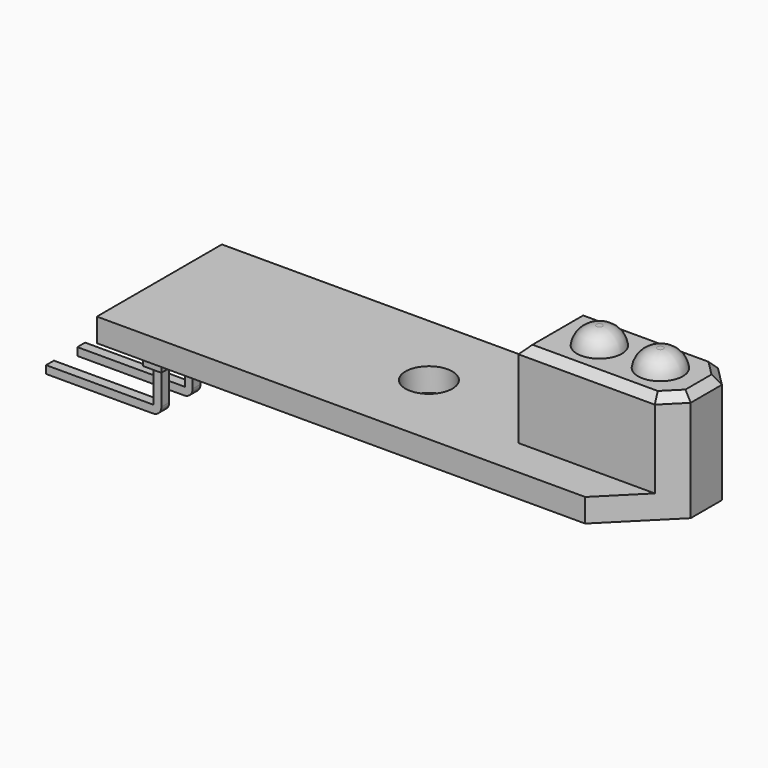
from build123d import *

# Parameters (mm, degrees)
F1_DEPTH  = 1.524
F3_DEPTH  = 5.588
F4_R      = 1.4605
F5_DEPTH  = 1.143
F7_SIZE   = 0.508
F9_DEPTH  = 0.3175
F12_W     = 1.2032650411
F12_H     = 6.585133262
F12_W_2   = 0.508
F12_H_2   = 0.635
F13_DEPTH = 1.524
F14_R     = 1.524
F15_DEPTH = 25.4


# Not quite as in the source:
# - a fillet or chamfer that OpenCascade refuses, or shapes differently, is made with other operations: its cross-section is extruded or revolved along the edge and cut away or added


with BuildPart() as f1:
    # F0 (on Top) → F1 (new body)
    with BuildSketch(Plane.XY):
        Polygon((-17.78, -5.08), (13.97, -5.08), (16.4832153797, -2.5667846203), (7.62, -2.5667846203), (7.62, 2.5667846203), (16.4832153797, 2.5667846203), (13.97, 5.08), (-17.78, 5.08), align=None)
        Polygon((7.62, -2.5667846203), (16.4832153797, -2.5667846203), (17.78, -1.27), (17.78, 1.27), (16.4832153797, 2.5667846203), (7.62, 2.5667846203), align=None)
    extrude(amount=-F1_DEPTH)

    # F2 (on face) → F3 (join)
    with BuildSketch(Plane.XY):
        Polygon((16.4832153797, -2.5667846203), (17.78, -1.27), (17.78, 1.27), (16.4832153797, 2.5667846203), (7.62, 2.5667846203), (7.62, -2.5667846203), align=None)
    extrude(amount=F3_DEPTH)

    # F4 (on face) → F5 (join)
    with BuildSketch(Plane.XY.offset(5.588)):
        with Locations((10.829353705, 0)):
            Circle(F4_R)
        with Locations((14.7973923013, 0)):
            Circle(F4_R)
    extrude(amount=F5_DEPTH)

    # F6: fillet of radius 1.27 on 2 edges, made by hand

    # F6_s1 → F6_t2 (revolve, cut)
    with BuildSketch(Plane.XZ):
        with BuildLine():
            ThreePointArc((12.289853705, 5.588), (11.8781615594, 6.4028572079), (11.0262196599, 6.731))
            Line((11.0262196599, 6.731), (12.289853705, 6.731))
            Line((12.289853705, 6.731), (12.289853705, 5.588))
        make_face()
    revolve(axis=Axis((10.829353705, 0, 6.731), (0, 0, 1)), mode=Mode.SUBTRACT)

    # F6_s3 → F6_t4 (revolve, cut)
    with BuildSketch(Plane.XZ):
        with BuildLine():
            ThreePointArc((16.2578923013, 5.588), (15.8462001556, 6.4028572079), (14.9942582561, 6.731))
            Line((14.9942582561, 6.731), (16.2578923013, 6.731))
            Line((16.2578923013, 6.731), (16.2578923013, 5.588))
        make_face()
    revolve(axis=Axis((14.7973923013, 0, 6.731), (0, 0, 1)), mode=Mode.SUBTRACT)

    # F7
    f7_edges = [f1.edges().sort_by_distance(p)[0] for p in [
        (12.051608, -2.566785, 5.588),
        (12.051608, 2.566785, 5.588),
        (7.62, 0, 5.588),
        (17.78, 0, 5.588),
        (17.131608, -1.918392, 5.588),
        (17.131608, 1.918392, 5.588),
    ]]
    chamfer(f7_edges, length=F7_SIZE)

    # F11: F10_1 across plane


with BuildPart() as f9:
    # F8 (on Front) → F9 (new body, symmetric)
    with BuildSketch(Plane.XZ):
        with BuildLine():
            Line((-22.86, -5.334), (-22.86, -5.842))
            Line((-22.86, -5.842), (-15.9157037269, -5.842))
            ThreePointArc((-15.9157037269, -5.842), (-15.5230394847, -5.6793531454), (-15.3603926301, -5.2866889032))
            Line((-15.3603926301, -5.2866889032), (-15.3603926301, -1.1672781548))
            Line((-15.3603926301, -1.1672781548), (-15.8683926301, -1.1672781548))
            Line((-15.8683926301, -1.1672781548), (-15.8683926301, -5.334))
            Line((-15.8683926301, -5.334), (-22.86, -5.334))
        make_face()
    extrude(amount=F9_DEPTH, both=True)


with BuildPart() as f10_1:
    # F10: copy of F9
    add(f9.part.moved(Location((0, -2.54, 0))))


with BuildPart() as f1_1:
    add(f1.part)
    add(f10_1.part.mirror(Plane.XZ))


    add(f9.part)  # F13 merges F9

    add(f10_1.part)  # F13 merges F10_1
    # F12 (on face) → F13 (join)
    with BuildSketch(Plane(origin=(0, 0, -1.524), x_dir=(1, 0, 0), z_dir=(0, 0, -1))):
        with Locations((-15.6205464154, 0)):
            Rectangle(F12_W, F12_H)
        with Locations((-15.6143926301, -2.54)):
            Rectangle(F12_W_2, F12_H_2, mode=Mode.SUBTRACT)
    extrude(amount=F13_DEPTH)

    # F14 (on face) → F15 (cut)
    with BuildSketch(Plane(origin=(0, 0, -1.524), x_dir=(1, 0, 0), z_dir=(0, 0, -1))):
        with Locations((-0.254, 0)):
            Circle(F14_R)
    extrude(amount=-F15_DEPTH, mode=Mode.SUBTRACT)


solid = f1_1.part
